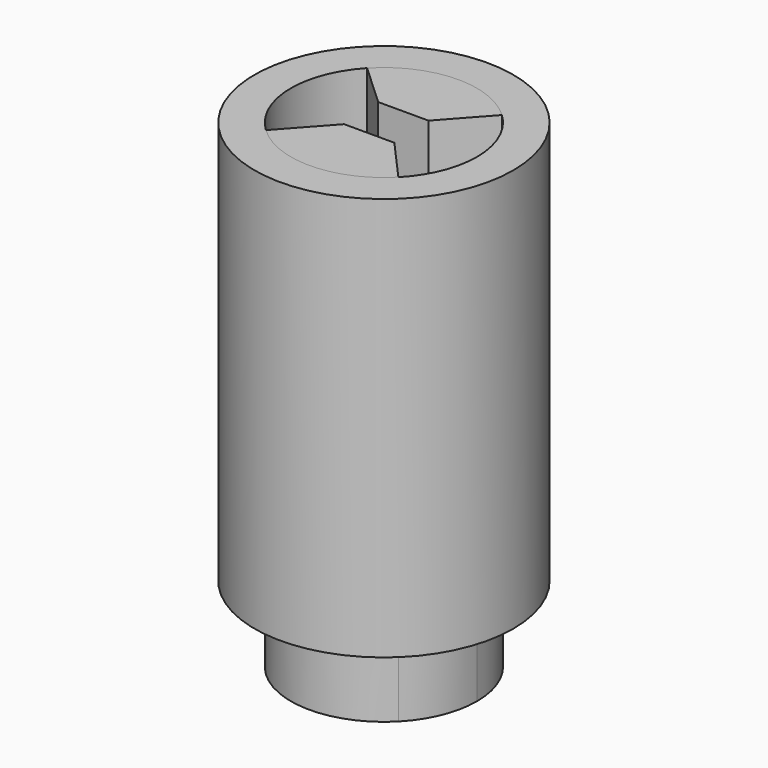
from build123d import *

# Parameters (mm, degrees)
F1_DEPTH = 15
F2_DEPTH = 15
F3_DEPTH = 80
F0_R     = 25.653928931
F4_DEPTH = 80


with BuildPart() as f1:
    # F0 (on Top) → F1 (new body)
    with BuildSketch(Plane.XY):
        with BuildLine():
            ThreePointArc((13.1836396394, -12.900506629), (17.0793508005, -6.9661468302), (18.4453632501, 0))
            ThreePointArc((18.4453632501, 0), (16.9458069689, 7.2849880988), (12.6909575623, 13.3854780108))
            Line((12.6909575623, 13.3854780108), (4.9841781147, 4.8152967356))
            Line((4.9841781147, 4.8152967356), (-4.9841781147, 4.8152967356))
            Line((-4.9841781147, 4.8152967356), (-13.4393265471, 12.6339197159))
            ThreePointArc((-13.4393265471, 12.6339197159), (-18.4374669621, -0.5396641983), (-12.6773625282, -13.398354554))
            Line((-12.6773625282, -13.398354554), (-4.4766523545, -4.2789067677))
            Line((-4.4766523545, -4.2789067677), (5.4917038749, -4.2789067677))
            Line((5.4917038749, -4.2789067677), (13.1836396394, -12.900506629))
        make_face()
    extrude(amount=F1_DEPTH)


with BuildPart() as f2:
    # F0 (on Top) → F2 (new body)
    with BuildSketch(Plane.XY):
        with BuildLine():
            Line((4.9841781147, 4.8152967356), (12.6909575623, 13.3854780108))
            ThreePointArc((12.6909575623, 13.3854780108), (-0.5303055742, 18.4377385117), (-13.4393265471, 12.6339197159))
            Line((-13.4393265471, 12.6339197159), (-4.9841781147, 4.8152967356))
            Line((-4.9841781147, 4.8152967356), (4.9841781147, 4.8152967356))
        make_face()
        with BuildLine():
            ThreePointArc((13.1836396394, -12.900506629), (17.0793508005, -6.9661468302), (18.4453632501, 0))
            ThreePointArc((18.4453632501, 0), (16.9458069689, 7.2849880988), (12.6909575623, 13.3854780108))
            Line((12.6909575623, 13.3854780108), (4.9841781147, 4.8152967356))
            Line((4.9841781147, 4.8152967356), (-4.9841781147, 4.8152967356))
            Line((-4.9841781147, 4.8152967356), (-13.4393265471, 12.6339197159))
            ThreePointArc((-13.4393265471, 12.6339197159), (-18.4374669621, -0.5396641983), (-12.6773625282, -13.398354554))
            Line((-12.6773625282, -13.398354554), (-4.4766523545, -4.2789067677))
            Line((-4.4766523545, -4.2789067677), (5.4917038749, -4.2789067677))
            Line((5.4917038749, -4.2789067677), (13.1836396394, -12.900506629))
        make_face()
        with BuildLine():
            ThreePointArc((-12.6773625282, -13.398354554), (0.3550243195, -18.4419462953), (13.1836396394, -12.900506629))
            Line((13.1836396394, -12.900506629), (5.4917038749, -4.2789067677))
            Line((5.4917038749, -4.2789067677), (-4.4766523545, -4.2789067677))
            Line((-4.4766523545, -4.2789067677), (-12.6773625282, -13.398354554))
        make_face()
    extrude(amount=-F2_DEPTH)

    # F0 (on Top) → F3 (join)
    with BuildSketch(Plane.XY):
        with BuildLine():
            ThreePointArc((-12.6773625282, -13.398354554), (0.3550243195, -18.4419462953), (13.1836396394, -12.900506629))
            Line((13.1836396394, -12.900506629), (5.4917038749, -4.2789067677))
            Line((5.4917038749, -4.2789067677), (-4.4766523545, -4.2789067677))
            Line((-4.4766523545, -4.2789067677), (-12.6773625282, -13.398354554))
        make_face()
        with BuildLine():
            Line((4.9841781147, 4.8152967356), (12.6909575623, 13.3854780108))
            ThreePointArc((12.6909575623, 13.3854780108), (-0.5303055742, 18.4377385117), (-13.4393265471, 12.6339197159))
            Line((-13.4393265471, 12.6339197159), (-4.9841781147, 4.8152967356))
            Line((-4.9841781147, 4.8152967356), (4.9841781147, 4.8152967356))
        make_face()
    extrude(amount=F3_DEPTH)


with BuildPart() as f4:
    # F0 (on Top) → F4 (new body)
    with BuildSketch(Plane.XY):
        Circle(F0_R)
        with BuildLine():
            ThreePointArc((12.6909575623, 13.3854780108), (16.9458069689, 7.2849880988), (18.4453632501, 0))
            ThreePointArc((18.4453632501, 0), (17.0793508005, -6.9661468302), (13.1836396394, -12.900506629))
            ThreePointArc((13.1836396394, -12.900506629), (0.3550243195, -18.4419462953), (-12.6773625282, -13.398354554))
            ThreePointArc((-12.6773625282, -13.398354554), (-18.4374669621, -0.5396641983), (-13.4393265471, 12.6339197159))
            ThreePointArc((-13.4393265471, 12.6339197159), (-0.5303055742, 18.4377385117), (12.6909575623, 13.3854780108))
        make_face(mode=Mode.SUBTRACT)
    extrude(amount=F4_DEPTH)


solid = Compound([f1.part, f2.part, f4.part])
